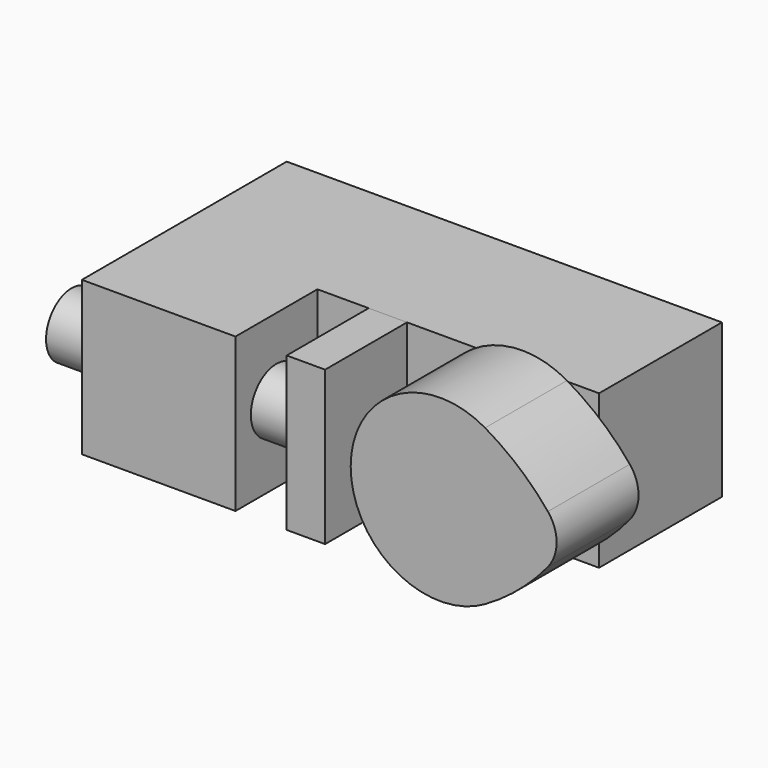
from build123d import *

# Parameters (mm, degrees)
F0_R          = 12.7
F1_DEPTH      = 25.4
F2_R          = 12.7
F3_DEPTH      = 25.4
F3_DEPTH_BACK = 38.1
F4_W          = 107.95
F4_H          = 38.1
F4_R          = 12.7
F5_DEPTH      = 38.1
F7_START      = -50.8
F6_W          = 25.4
F6_H          = 38.1
F6_R          = 7.9375
F7_DEPTH      = 38.1
F8_START      = -28.575
F8_DEPTH      = 9.525
F10_START     = -28.575
F9_R          = 7.9375
F10_DEPTH     = 73.025


with BuildPart() as f1:
    # F0 (on Front) → F1 (new body)
    with BuildSketch(Plane.XZ):
        with BuildLine():
            ThreePointArc((26.682561162, 6.0491874454), (19.4915271669, 13.3490438618), (11.1125, 19.2474145991))
            ThreePointArc((11.1125, 19.2474145991), (-22.225, 0), (11.1125, -19.2474145991))
            ThreePointArc((11.1125, -19.2474145991), (19.4915271669, -13.3490438618), (26.682561162, -6.0491874454))
            ThreePointArc((26.682561162, -6.0491874454), (28.8500509684, 0), (26.682561162, 6.0491874454))
        make_face()
        Circle(F0_R, mode=Mode.SUBTRACT)
    extrude(amount=F1_DEPTH)

    # F2 (on Front) → F3 (join, two sides)
    with BuildSketch(Plane.XZ) as f3_sk:
        Circle(F2_R)
    extrude(amount=F3_DEPTH)
    extrude(f3_sk.sketch, amount=-F3_DEPTH_BACK)


with BuildPart() as f5:
    # F4 (on Front) → F5 (new body)
    with BuildSketch(Plane.XZ):
        with Locations((-34.925, 0)):
            Rectangle(F4_W, F4_H)
        Circle(F4_R, mode=Mode.SUBTRACT)
    extrude(amount=-F5_DEPTH)

    # F6 (on Right) → F7 (join)
    with BuildSketch(Plane.YZ.offset(F7_START)):
        with Locations((-12.7, 0)):
            Rectangle(F6_W, F6_H)
        with Locations((-12.7, 0)):
            Circle(F6_R, mode=Mode.SUBTRACT)
    extrude(amount=-F7_DEPTH)


with BuildPart() as f8:
    # F6 (on Right) → F8 (new body)
    with BuildSketch(Plane.YZ.offset(F8_START)):
        with Locations((-12.7, 0)):
            Rectangle(F6_W, F6_H)
        with Locations((-12.7, 0)):
            Circle(F6_R, mode=Mode.SUBTRACT)
    extrude(amount=-F8_DEPTH)

    # F9 (on Right) → F10 (join)
    with BuildSketch(Plane.YZ.offset(F10_START)):
        with Locations((-12.7, 0)):
            Circle(F9_R)
    extrude(amount=-F10_DEPTH)


solid = Compound([f1.part, f5.part, f8.part])
